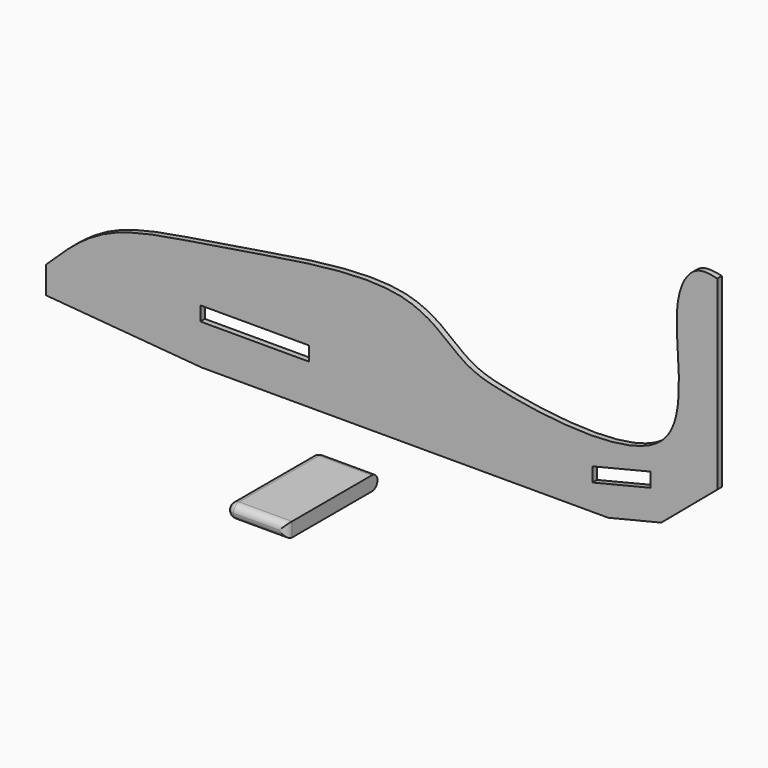
from build123d import *

# Parameters (mm, degrees)
F0_W     = 76.2
F0_H     = 10
F1_DEPTH = 4
F2_W     = 42
F2_H     = 10
F3_DEPTH = 80
F4_R     = 4.99999


# Not quite as in the source:
# - a fillet or chamfer is up to 0.001 mm smaller than in the source, because OpenCascade refuses the exact size


with BuildPart() as f1:
    # F0 (on Front) → F1 (new body)
    with BuildSketch(Plane.XZ):
        with BuildLine():
            add(Edge.make_bspline(
                [(-231.6725862107, 0), (-219.0993671328, 12.343248795), (-190.5459015942, 40.3744575823), (-107.4143479778, 48.8125552497), (19.6408862931, 75.2535030954), (58.229683436, 34.3949690879), (88.1193610303, 23.6775246845), (231.2402117739, 5.043023493), (202.5783639872, 115.4317400021), (221.4998393715, 148.0646570715), (233.9718904053, 145.4679123311), (239.0467838633, 144.4112935873)],
                knots=[0, 0, 0, 0, 0.1046742923, 0.2377126956, 0.3989739008, 0.4962321415, 0.5817787109, 0.7323531864, 0.8642732523, 0.9447726134, 1, 1, 1, 1], degree=3))
            Line((-231.6725862107, 0), (-231.6725862107, -19.0499990361))
            Line((-231.6725862107, -19.0499990361), (-122.4797673147, -28.1355770861))
            Line((-122.4797673147, -28.1355770861), (127.0137888456, -28.1355770861))
            Line((127.0137888456, -28.1355770861), (162.6557133227, -28.1355770861))
            Line((162.6557133227, -28.1355770861), (199.717745138, -19.0499990361))
            Line((199.717745138, -19.0499990361), (239.0467838633, 14.1338711232))
            Line((239.0467838633, 14.1338711232), (239.0467838633, 144.4112935873))
        make_face()
        with Locations((-85.4177412825, 5)):
            Rectangle(F0_W, F0_H, mode=Mode.SUBTRACT)
        Polygon((151.428103447, -10), (151.428103447, 0), (192.2202595557, 10), (192.2202595557, 0), align=None, mode=Mode.SUBTRACT)
    extrude(amount=F1_DEPTH)


with BuildPart() as f3:
    # F2 (on Front) → F3 (new body)
    with BuildSketch(Plane.XZ):
        with Locations((-23.4696671832, -60.190187508)):
            Rectangle(F2_W, F2_H)
    extrude(amount=F3_DEPTH)

    # F4 (radius 5 in the source; OpenCascade refuses exactly that, so slightly less here)
    f4_edges = [f3.edges().sort_by_distance(p)[0] for p in [
        (-44.469667, -40, -55.190188),
        (-44.469667, -40, -65.190188),
        (-44.469667, -80, -60.190188),
        (-44.469667, 0, -60.190188),
        (-23.469667, -80, -55.190188),
        (-23.469667, -80, -65.190188),
        (-2.469667, -80, -60.190188),
        (-23.469667, 0, -55.190188),
        (-23.469667, 0, -65.190188),
    ]]
    fillet(f4_edges, radius=F4_R)


solid = Compound([f1.part, f3.part])
